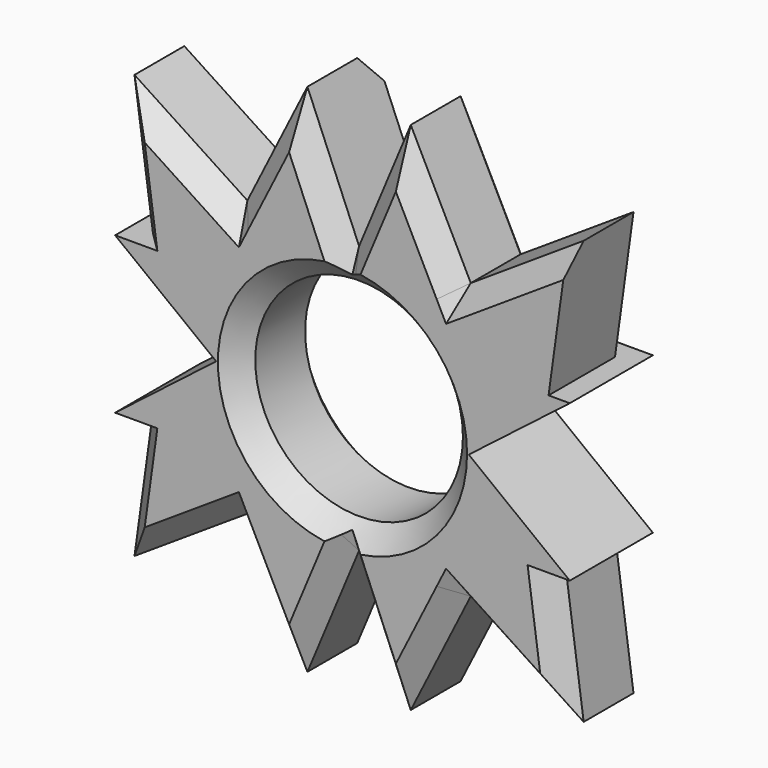
from build123d import *

# Parameters (mm, degrees)
F0_R          = 25.4053922475
F1_DEPTH      = 25.4
F2_SIZE       = 5.08
F3_T4_DEPTH   = 58.8942991577
F3_T9_DEPTH   = 59.1482991577
F3_T14_DEPTH  = 59.1482991577
F3_T19_DEPTH  = 59.1482991577
F3_T24_DEPTH  = 59.1482991577
F3_T29_DEPTH  = 58.8942991577
F3_T34_DEPTH  = 58.8942991577
F3_T39_DEPTH  = 58.8942991577
F3_T44_DEPTH  = 58.8942991577
F3_T49_DEPTH  = 59.1482991577
F3_T54_DEPTH  = 59.1482991577
F3_T59_DEPTH  = 58.8942991577
F3_T64_DEPTH  = 58.8942991577
F3_T69_DEPTH  = 59.1482991577
F3_T74_DEPTH  = 59.1482991577
F3_T79_DEPTH  = 59.1482991577
F3_T84_DEPTH  = 59.1482991577
F3_T89_DEPTH  = 58.8942991577
F3_T94_DEPTH  = 58.8942991577
F3_T99_DEPTH  = 58.8942991577
F3_T104_DEPTH = 59.1482991577
F3_T109_DEPTH = 59.1482991577
F3_T114_DEPTH = 59.1482991577
F3_T119_DEPTH = 58.8942991577
F3_T124_DEPTH = 59.1482991577
F3_T129_DEPTH = 59.1482991577
F3_T134_DEPTH = 58.8942991577
F3_T139_DEPTH = 58.8942991577
F3_T144_DEPTH = 58.8942991577
F3_T149_DEPTH = 58.8942991577


# Not quite as in the source:
# - a fillet or chamfer that OpenCascade refuses, or shapes differently, is made with other operations: its cross-section is extruded or revolved along the edge and cut away or added


with BuildPart() as f1:
    # F0 (on Front) → F1 (new body)
    with BuildSketch(Plane.XZ):
        Polygon((-55.6186027825, 19.1091839224), (-30.8941560641, 0), (-50.4200380058, 19.1091839224), align=None)
        Polygon((-54.9483810148, 51.8172029635), (-50.4200380058, 19.1091839224), (-27.3260947604, 33.7249476569), align=None)
        Polygon((-12.64267964, 63.0167225502), (-27.3260947604, 33.7249476569), (0, 32.7880373733), align=None)
        Polygon((12.64267964, 63.0167225502), (0, 32.7880373733), (27.3260947604, 33.7249476569), align=None)
        Polygon((54.9483810148, 51.8172029635), (27.3260947604, 33.7249476569), (50.4200380058, 19.1091839224), align=None)
        Polygon((55.6186027825, 19.1091839224), (50.4200380058, 19.1091839224), (30.8941560641, 0), align=None)
        Polygon((0, -32.7880373733), (-27.3260947604, -33.7249476569), (-12.64267964, -63.0167225502), align=None)
        Polygon((-27.3260947604, -33.7249476569), (-50.4200380058, -19.1091839224), (-54.9483810148, -51.8172029635), align=None)
        Polygon((-50.4200380058, -19.1091839224), (-30.8941560641, 0), (-55.6186027825, -19.1091839224), align=None)
        Polygon((27.3260947604, -33.7249476569), (0, -32.7880373733), (12.64267964, -63.0167225502), align=None)
        Polygon((50.4200380058, -19.1091839224), (27.3260947604, -33.7249476569), (54.9483810148, -51.8172029635), align=None)
        Polygon((30.8941560641, 0), (50.4200380058, -19.1091839224), (55.6186027825, -19.1091839224), align=None)
        Polygon((-50.4200380058, 19.1091839224), (-30.8941560641, 0), (-50.4200380058, -19.1091839224), (-27.3260947604, -33.7249476569), (0, -32.7880373733), (27.3260947604, -33.7249476569), (50.4200380058, -19.1091839224), (30.8941560641, 0), (50.4200380058, 19.1091839224), (27.3260947604, 33.7249476569), (0, 32.7880373733), (-27.3260947604, 33.7249476569), align=None)
        Circle(F0_R, mode=Mode.SUBTRACT)
    extrude(amount=F1_DEPTH)

    # F2
    f2_edges = [f1.edges().sort_by_distance(p)[0] for p in [
        (-25.405392, 0, 0),
        (-25.405392, -25.4, 0),
    ]]
    chamfer(f2_edges, length=F2_SIZE)

    # F3: chamfer of 5.08 on 30 edges, made by hand


with BuildPart() as f3_tool2:
    # F3_s3 → F3_t4 (new body)
    with BuildSketch(Plane(origin=(28.5608965027, 0, 56.9758018995), x_dir=(0, 1, 0), z_dir=(-0.4481296197, 0, -0.8939685922))):
        Polygon((0, -34.4618184336), (-5.08, -39.5418184336), (0, -39.5418184336), align=None)
    extrude(amount=F3_T4_DEPTH)

    split(bisect_by=Plane(origin=(2.2353786575, 4.079767946, 3.4128563917), x_dir=(-0.8769857612, 0.4805163626, 0), z_dir=(0.3874365964, 0.7071067812, 0.5915174416)), keep=Keep.TOP)


with BuildPart() as f1_1:
    add(f1.part)

    # F3_t1: cut F3_tool2
    add(f3_tool2.part, mode=Mode.SUBTRACT)


with BuildPart() as f3_tool7:
    # F3_s8 → F3_t9 (new body)
    with BuildSketch(Plane(origin=(-23.6516969458, 0, 15.4915684979), x_dir=(0, 1, 0), z_dir=(-0.8365319883, 0, 0.5479180892))):
        Polygon((0, -8.159535892), (-5.08, -13.239535892), (0, -13.239535892), align=None)
    extrude(amount=F3_T9_DEPTH)

    split(bisect_by=Plane(origin=(-15.4038916556, 17.2309092168, 7.7216807951), x_dir=(-0.7455258584, -0.6664767021, 0), z_dir=(-0.6321312537, 0.7071067812, 0.316875493)), keep=Keep.TOP)


with BuildPart() as f1_2:
    add(f1_1.part)

    # F3_t6: cut F3_tool7
    add(f3_tool7.part, mode=Mode.SUBTRACT)


with BuildPart() as f3_tool12:
    # F3_s13 → F3_t14 (new body)
    with BuildSketch(Plane(origin=(-9.8640749157, 0, 71.247771982), x_dir=(0, 1, 0), z_dir=(0.1371394006, 0, -0.9905517578))):
        Polygon((0, -42.2430352429), (-5.08, -47.3230352429), (0, -47.3230352429), align=None)
    extrude(amount=F3_T14_DEPTH)

    split(bisect_by=Plane.XY.offset(19.1091839224), keep=Keep.TOP)


with BuildPart() as f1_3:
    add(f1_2.part)

    # F3_t11: cut F3_tool12
    add(f3_tool12.part, mode=Mode.SUBTRACT)


with BuildPart() as f3_tool17:
    # F3_s18 → F3_t19 (new body)
    with BuildSketch(Plane(origin=(-1.7525126205, 0, -12.658320283), x_dir=(0, 1, 0), z_dir=(-0.1371394006, 0, -0.9905517578))):
        Polygon((0, -42.2430352429), (-5.08, -47.3230352429), (0, -47.3230352429), align=None)
    extrude(amount=F3_T19_DEPTH)

    split(bisect_by=Plane.XY.offset(-19.1091839224), keep=Keep.BOTTOM)


with BuildPart() as f1_4:
    add(f1_3.part)

    # F3_t16: cut F3_tool17
    add(f3_tool17.part, mode=Mode.SUBTRACT)


with BuildPart() as f3_tool22:
    # F3_s23 → F3_t24 (new body)
    with BuildSketch(Plane(origin=(-73.1311412461, 0, -47.8999915541), x_dir=(0, 1, 0), z_dir=(0.8365319883, 0, 0.5479180892))):
        Polygon((0, -8.159535892), (-5.08, -13.239535892), (0, -13.239535892), align=None)
    extrude(amount=F3_T24_DEPTH)

    split(bisect_by=Plane(origin=(-15.4038916556, 17.2309092168, -7.7216807951), x_dir=(-0.7455258584, -0.6664767021, 0), z_dir=(-0.6321312537, 0.7071067812, -0.316875493)), keep=Keep.TOP)


with BuildPart() as f1_5:
    add(f1_4.part)

    # F3_t21: cut F3_tool22
    add(f3_tool22.part, mode=Mode.SUBTRACT)


with BuildPart() as f3_tool27:
    # F3_s28 → F3_t29 (new body)
    with BuildSketch(Plane(origin=(2.1686166163, 0, -4.3261481905), x_dir=(0, 1, 0), z_dir=(0.4481296197, 0, -0.8939685922))):
        Polygon((0, -34.4618184336), (-5.08, -39.5418184336), (0, -39.5418184336), align=None)
    extrude(amount=F3_T29_DEPTH)

    split(bisect_by=Plane(origin=(2.2353786575, 4.079767946, -3.4128563917), x_dir=(-0.8769857612, 0.4805163626, 0), z_dir=(0.3874365964, 0.7071067812, -0.5915174416)), keep=Keep.TOP)


with BuildPart() as f1_6:
    add(f1_5.part)

    # F3_t26: cut F3_tool27
    add(f3_tool27.part, mode=Mode.SUBTRACT)


with BuildPart() as f3_tool32:
    # F3_s33 → F3_t34 (new body)
    with BuildSketch(Plane(origin=(-29.3549569097, 0, -70.1877905691), x_dir=(0, 1, 0), z_dir=(0.3858475139, 0, 0.9225625703))):
        Polygon((0, -7.5711827057), (-5.08, -12.6511827057), (0, -12.6511827057), align=None)
    extrude(amount=F3_T34_DEPTH)

    split(bisect_by=Plane(origin=(-3.4924448884, 3.7855913528, -1.4606610121), x_dir=(-0.7349918349, -0.6780759564, 0), z_dir=(-0.6523502495, 0.7071067812, -0.2728353936)), keep=Keep.TOP)


with BuildPart() as f1_7:
    add(f1_6.part)

    # F3_t31: cut F3_tool32
    add(f3_tool32.part, mode=Mode.SUBTRACT)


with BuildPart() as f3_tool37:
    # F3_s38 → F3_t39 (new body)
    with BuildSketch(Plane(origin=(6.6307379976, 0, -15.854114565), x_dir=(0, 1, 0), z_dir=(0.3858475139, 0, -0.9225625703))):
        Polygon((0, -7.5711827057), (-5.08, -12.6511827057), (0, -12.6511827057), align=None)
    extrude(amount=F3_T39_DEPTH)

    split(bisect_by=Plane(origin=(3.4924448884, 3.7855913528, -1.4606610121), x_dir=(-0.7349918349, 0.6780759564, 0), z_dir=(0.6523502495, 0.7071067812, -0.2728353936)), keep=Keep.TOP)


with BuildPart() as f1_8:
    add(f1_7.part)

    # F3_t36: cut F3_tool37
    add(f3_tool37.part, mode=Mode.SUBTRACT)


with BuildPart() as f3_tool42:
    # F3_s43 → F3_t44 (new body)
    with BuildSketch(Plane(origin=(-28.5608965027, 0, -56.9758018995), x_dir=(0, 1, 0), z_dir=(0.4481296197, 0, 0.8939685922))):
        Polygon((0, -34.4618184336), (-5.08, -39.5418184336), (0, -39.5418184336), align=None)
    extrude(amount=F3_T44_DEPTH)

    split(bisect_by=Plane(origin=(-2.2353786575, 4.079767946, -3.4128563917), x_dir=(-0.8769857612, -0.4805163626, 0), z_dir=(-0.3874365964, 0.7071067812, -0.5915174416)), keep=Keep.TOP)


with BuildPart() as f1_9:
    add(f1_8.part)

    # F3_t41: cut F3_tool42
    add(f3_tool42.part, mode=Mode.SUBTRACT)


with BuildPart() as f3_tool47:
    # F3_s48 → F3_t49 (new body)
    with BuildSketch(Plane(origin=(23.6516969458, 0, -15.4915684979), x_dir=(0, 1, 0), z_dir=(0.8365319883, 0, -0.5479180892))):
        Polygon((0, -8.159535892), (-5.08, -13.239535892), (0, -13.239535892), align=None)
    extrude(amount=F3_T49_DEPTH)

    split(bisect_by=Plane(origin=(15.4038916556, 17.2309092168, -7.7216807951), x_dir=(-0.7455258584, 0.6664767021, 0), z_dir=(0.6321312537, 0.7071067812, -0.316875493)), keep=Keep.TOP)


with BuildPart() as f1_10:
    add(f1_9.part)

    # F3_t46: cut F3_tool47
    add(f3_tool47.part, mode=Mode.SUBTRACT)


with BuildPart() as f3_tool52:
    # F3_s53 → F3_t54 (new body)
    with BuildSketch(Plane(origin=(9.8640749157, 0, -71.247771982), x_dir=(0, 1, 0), z_dir=(-0.1371394006, 0, 0.9905517578))):
        Polygon((0, -42.2430352429), (-5.08, -47.3230352429), (0, -47.3230352429), align=None)
    extrude(amount=F3_T54_DEPTH)

    split(bisect_by=Plane.XY.offset(-19.1091839224), keep=Keep.BOTTOM)


with BuildPart() as f1_11:
    add(f1_10.part)

    # F3_t51: cut F3_tool52
    add(f3_tool52.part, mode=Mode.SUBTRACT)


with BuildPart() as f3_tool57:
    # F3_s58 → F3_t59 (new body)
    with BuildSketch(Plane(origin=(29.3549569097, 0, 70.1877905691), x_dir=(0, 1, 0), z_dir=(-0.3858475139, 0, -0.9225625703))):
        Polygon((0, -7.5711827057), (-5.08, -12.6511827057), (0, -12.6511827057), align=None)
    extrude(amount=F3_T59_DEPTH)

    split(bisect_by=Plane(origin=(11.6715076337, 0, 4.8814273947), x_dir=(0, 1, 0), z_dir=(0.9225625703, 0, 0.3858475139)), keep=Keep.TOP)


with BuildPart() as f1_12:
    add(f1_11.part)

    # F3_t56: cut F3_tool57
    add(f3_tool57.part, mode=Mode.SUBTRACT)


with BuildPart() as f3_tool62:
    # F3_s63 → F3_t64 (new body)
    with BuildSketch(Plane(origin=(-2.1686166163, 0, 4.3261481905), x_dir=(0, 1, 0), z_dir=(-0.4481296197, 0, 0.8939685922))):
        Polygon((0, -34.4618184336), (-5.08, -39.5418184336), (0, -39.5418184336), align=None)
    extrude(amount=F3_T64_DEPTH)

    split(bisect_by=Plane(origin=(-2.2353786575, 4.079767946, 3.4128563917), x_dir=(-0.8769857612, -0.4805163626, 0), z_dir=(-0.3874365964, 0.7071067812, 0.5915174416)), keep=Keep.TOP)


with BuildPart() as f1_13:
    add(f1_12.part)

    # F3_t61: cut F3_tool62
    add(f3_tool62.part, mode=Mode.SUBTRACT)


with BuildPart() as f3_tool67:
    # F3_s68 → F3_t69 (new body)
    with BuildSketch(Plane(origin=(73.1311412461, 0, 47.8999915541), x_dir=(0, 1, 0), z_dir=(-0.8365319883, 0, -0.5479180892))):
        Polygon((0, -8.159535892), (-5.08, -13.239535892), (0, -13.239535892), align=None)
    extrude(amount=F3_T69_DEPTH)

    split(bisect_by=Plane(origin=(15.4038916556, 17.2309092168, 7.7216807951), x_dir=(-0.7455258584, 0.6664767021, 0), z_dir=(0.6321312537, 0.7071067812, 0.316875493)), keep=Keep.TOP)


with BuildPart() as f1_14:
    add(f1_13.part)

    # F3_t66: cut F3_tool67
    add(f3_tool67.part, mode=Mode.SUBTRACT)


with BuildPart() as f3_tool72:
    # F3_s73 → F3_t74 (new body)
    with BuildSketch(Plane(origin=(1.7525126205, 0, 12.658320283), x_dir=(0, 1, 0), z_dir=(0.1371394006, 0, 0.9905517578))):
        Polygon((0, -42.2430352429), (-5.08, -47.3230352429), (0, -47.3230352429), align=None)
    extrude(amount=F3_T74_DEPTH)

    split(bisect_by=Plane.XY.offset(19.1091839224), keep=Keep.TOP)


with BuildPart() as f1_15:
    add(f1_14.part)

    # F3_t71: cut F3_tool72
    add(f3_tool72.part, mode=Mode.SUBTRACT)


with BuildPart() as f3_tool77:
    # F3_s78 → F3_t79 (new body)
    with BuildSketch(Plane(origin=(-9.8640749157, 0, 71.247771982), x_dir=(0, 1, 0), z_dir=(0.1371394006, 0, -0.9905517578))):
        Polygon((-25.4, -42.2430352429), (-20.32, -47.3230352429), (-25.4, -47.3230352429), align=None)
    extrude(amount=F3_T79_DEPTH)

    split(bisect_by=Plane.XY.offset(19.1091839224), keep=Keep.TOP)


with BuildPart() as f1_16:
    add(f1_15.part)

    # F3_t76: cut F3_tool77
    add(f3_tool77.part, mode=Mode.SUBTRACT)


with BuildPart() as f3_tool82:
    # F3_s83 → F3_t84 (new body)
    with BuildSketch(Plane(origin=(-23.6516969458, 0, 15.4915684979), x_dir=(0, 1, 0), z_dir=(-0.8365319883, 0, 0.5479180892))):
        Polygon((-25.4, -8.159535892), (-20.32, -13.239535892), (-25.4, -13.239535892), align=None)
    extrude(amount=F3_T84_DEPTH)

    split(bisect_by=Plane(origin=(-26.757292777, -29.9309092168, 13.4129269658), x_dir=(0.7455258584, -0.6664767021, 0), z_dir=(-0.6321312537, -0.7071067812, 0.316875493)), keep=Keep.TOP)


with BuildPart() as f1_17:
    add(f1_16.part)

    # F3_t81: cut F3_tool82
    add(f3_tool82.part, mode=Mode.SUBTRACT)


with BuildPart() as f3_tool87:
    # F3_s88 → F3_t89 (new body)
    with BuildSketch(Plane(origin=(28.5608965027, 0, 56.9758018995), x_dir=(0, 1, 0), z_dir=(-0.4481296197, 0, -0.8939685922))):
        Polygon((-25.4, -34.4618184336), (-20.32, -39.5418184336), (-25.4, -39.5418184336), align=None)
    extrude(amount=F3_T89_DEPTH)

    split(bisect_by=Plane(origin=(9.1939383908, -16.779767946, 14.0368126434), x_dir=(0.8769857612, 0.4805163626, 0), z_dir=(0.3874365964, -0.7071067812, 0.5915174416)), keep=Keep.TOP)


with BuildPart() as f1_18:
    add(f1_17.part)

    # F3_t86: cut F3_tool87
    add(f3_tool87.part, mode=Mode.SUBTRACT)


with BuildPart() as f3_tool92:
    # F3_s93 → F3_t94 (new body)
    with BuildSketch(Plane(origin=(-6.6307379976, 0, 15.854114565), x_dir=(0, 1, 0), z_dir=(-0.3858475139, 0, 0.9225625703))):
        Polygon((-25.4, -7.5711827057), (-20.32, -12.6511827057), (-25.4, -12.6511827057), align=None)
    extrude(amount=F3_T94_DEPTH)

    split(bisect_by=Plane(origin=(-15.2089895306, -16.4855913528, 6.3609244384), x_dir=(0.7349918349, -0.6780759564, 0), z_dir=(-0.6523502495, -0.7071067812, 0.2728353936)), keep=Keep.TOP)


with BuildPart() as f1_19:
    add(f1_18.part)

    # F3_t91: cut F3_tool92
    add(f3_tool92.part, mode=Mode.SUBTRACT)


with BuildPart() as f3_tool97:
    # F3_s98 → F3_t99 (new body)
    with BuildSketch(Plane(origin=(29.3549569097, 0, 70.1877905691), x_dir=(0, 1, 0), z_dir=(-0.3858475139, 0, -0.9225625703))):
        Polygon((-25.4, -7.5711827057), (-20.32, -12.6511827057), (-25.4, -12.6511827057), align=None)
    extrude(amount=F3_T99_DEPTH)

    split(bisect_by=Plane(origin=(15.2089895306, -16.4855913528, 6.3609244384), x_dir=(0.7349918349, 0.6780759564, 0), z_dir=(0.6523502495, -0.7071067812, 0.2728353936)), keep=Keep.TOP)


with BuildPart() as f1_20:
    add(f1_19.part)

    # F3_t96: cut F3_tool97
    add(f3_tool97.part, mode=Mode.SUBTRACT)


with BuildPart() as f3_tool102:
    # F3_s103 → F3_t104 (new body)
    with BuildSketch(Plane(origin=(73.1311412461, 0, 47.8999915541), x_dir=(0, 1, 0), z_dir=(-0.8365319883, 0, -0.5479180892))):
        Polygon((-25.4, -8.159535892), (-20.32, -13.239535892), (-25.4, -13.239535892), align=None)
    extrude(amount=F3_T104_DEPTH)

    split(bisect_by=Plane(origin=(26.757292777, -29.9309092168, 13.4129269658), x_dir=(0.7455258584, 0.6664767021, 0), z_dir=(0.6321312537, -0.7071067812, 0.316875493)), keep=Keep.TOP)


with BuildPart() as f1_21:
    add(f1_20.part)

    # F3_t101: cut F3_tool102
    add(f3_tool102.part, mode=Mode.SUBTRACT)


with BuildPart() as f3_tool107:
    # F3_s108 → F3_t109 (new body)
    with BuildSketch(Plane(origin=(9.8640749157, 0, -71.247771982), x_dir=(0, 1, 0), z_dir=(-0.1371394006, 0, 0.9905517578))):
        Polygon((-25.4, -42.2430352429), (-20.32, -47.3230352429), (-25.4, -47.3230352429), align=None)
    extrude(amount=F3_T109_DEPTH)

    split(bisect_by=Plane.XY.offset(-19.1091839224), keep=Keep.BOTTOM)


with BuildPart() as f1_22:
    add(f1_21.part)

    # F3_t106: cut F3_tool107
    add(f3_tool107.part, mode=Mode.SUBTRACT)


with BuildPart() as f3_tool112:
    # F3_s113 → F3_t114 (new body)
    with BuildSketch(Plane(origin=(23.6516969458, 0, -15.4915684979), x_dir=(0, 1, 0), z_dir=(0.8365319883, 0, -0.5479180892))):
        Polygon((-25.4, -8.159535892), (-20.32, -13.239535892), (-25.4, -13.239535892), align=None)
    extrude(amount=F3_T114_DEPTH)

    split(bisect_by=Plane(origin=(26.757292777, -29.9309092168, -13.4129269658), x_dir=(0.7455258584, 0.6664767021, 0), z_dir=(0.6321312537, -0.7071067812, -0.316875493)), keep=Keep.TOP)


with BuildPart() as f1_23:
    add(f1_22.part)

    # F3_t111: cut F3_tool112
    add(f3_tool112.part, mode=Mode.SUBTRACT)


with BuildPart() as f3_tool117:
    # F3_s118 → F3_t119 (new body)
    with BuildSketch(Plane(origin=(-2.1686166163, 0, 4.3261481905), x_dir=(0, 1, 0), z_dir=(-0.4481296197, 0, 0.8939685922))):
        Polygon((-25.4, -34.4618184336), (-20.32, -39.5418184336), (-25.4, -39.5418184336), align=None)
    extrude(amount=F3_T119_DEPTH)

    split(bisect_by=Plane(origin=(-9.1939383908, -16.779767946, 14.0368126434), x_dir=(0.8769857612, -0.4805163626, 0), z_dir=(-0.3874365964, -0.7071067812, 0.5915174416)), keep=Keep.TOP)


with BuildPart() as f1_24:
    add(f1_23.part)

    # F3_t116: cut F3_tool117
    add(f3_tool117.part, mode=Mode.SUBTRACT)


with BuildPart() as f3_tool122:
    # F3_s123 → F3_t124 (new body)
    with BuildSketch(Plane(origin=(-1.7525126205, 0, -12.658320283), x_dir=(0, 1, 0), z_dir=(-0.1371394006, 0, -0.9905517578))):
        Polygon((-25.4, -42.2430352429), (-20.32, -47.3230352429), (-25.4, -47.3230352429), align=None)
    extrude(amount=F3_T124_DEPTH)

    split(bisect_by=Plane.XY.offset(-19.1091839224), keep=Keep.BOTTOM)


with BuildPart() as f1_25:
    add(f1_24.part)

    # F3_t121: cut F3_tool122
    add(f3_tool122.part, mode=Mode.SUBTRACT)


with BuildPart() as f3_tool127:
    # F3_s128 → F3_t129 (new body)
    with BuildSketch(Plane(origin=(-73.1311412461, 0, -47.8999915541), x_dir=(0, 1, 0), z_dir=(0.8365319883, 0, 0.5479180892))):
        Polygon((-25.4, -8.159535892), (-20.32, -13.239535892), (-25.4, -13.239535892), align=None)
    extrude(amount=F3_T129_DEPTH)

    split(bisect_by=Plane(origin=(-26.757292777, -29.9309092168, -13.4129269658), x_dir=(0.7455258584, -0.6664767021, 0), z_dir=(-0.6321312537, -0.7071067812, -0.316875493)), keep=Keep.TOP)


with BuildPart() as f1_26:
    add(f1_25.part)

    # F3_t126: cut F3_tool127
    add(f3_tool127.part, mode=Mode.SUBTRACT)


with BuildPart() as f3_tool132:
    # F3_s133 → F3_t134 (new body)
    with BuildSketch(Plane(origin=(2.1686166163, 0, -4.3261481905), x_dir=(0, 1, 0), z_dir=(0.4481296197, 0, -0.8939685922))):
        Polygon((-25.4, -34.4618184336), (-20.32, -39.5418184336), (-25.4, -39.5418184336), align=None)
    extrude(amount=F3_T134_DEPTH)

    split(bisect_by=Plane(origin=(9.1939383908, -16.779767946, -14.0368126434), x_dir=(0.8769857612, 0.4805163626, 0), z_dir=(0.3874365964, -0.7071067812, -0.5915174416)), keep=Keep.TOP)


with BuildPart() as f1_27:
    add(f1_26.part)

    # F3_t131: cut F3_tool132
    add(f3_tool132.part, mode=Mode.SUBTRACT)


with BuildPart() as f3_tool137:
    # F3_s138 → F3_t139 (new body)
    with BuildSketch(Plane(origin=(6.6307379976, 0, -15.854114565), x_dir=(0, 1, 0), z_dir=(0.3858475139, 0, -0.9225625703))):
        Polygon((-25.4, -7.5711827057), (-20.32, -12.6511827057), (-25.4, -12.6511827057), align=None)
    extrude(amount=F3_T139_DEPTH)

    split(bisect_by=Plane(origin=(15.2089895306, -16.4855913528, -6.3609244384), x_dir=(0.7349918349, 0.6780759564, 0), z_dir=(0.6523502495, -0.7071067812, -0.2728353936)), keep=Keep.TOP)


with BuildPart() as f1_28:
    add(f1_27.part)

    # F3_t136: cut F3_tool137
    add(f3_tool137.part, mode=Mode.SUBTRACT)


with BuildPart() as f3_tool142:
    # F3_s143 → F3_t144 (new body)
    with BuildSketch(Plane(origin=(-28.5608965027, 0, -56.9758018995), x_dir=(0, 1, 0), z_dir=(0.4481296197, 0, 0.8939685922))):
        Polygon((-25.4, -34.4618184336), (-20.32, -39.5418184336), (-25.4, -39.5418184336), align=None)
    extrude(amount=F3_T144_DEPTH)

    split(bisect_by=Plane(origin=(-9.1939383908, -16.779767946, -14.0368126434), x_dir=(0.8769857612, -0.4805163626, 0), z_dir=(-0.3874365964, -0.7071067812, -0.5915174416)), keep=Keep.TOP)


with BuildPart() as f1_29:
    add(f1_28.part)

    # F3_t141: cut F3_tool142
    add(f3_tool142.part, mode=Mode.SUBTRACT)


with BuildPart() as f3_tool147:
    # F3_s148 → F3_t149 (new body)
    with BuildSketch(Plane(origin=(-29.3549569097, 0, -70.1877905691), x_dir=(0, 1, 0), z_dir=(0.3858475139, 0, 0.9225625703))):
        Polygon((-25.4, -7.5711827057), (-20.32, -12.6511827057), (-25.4, -12.6511827057), align=None)
    extrude(amount=F3_T149_DEPTH)

    split(bisect_by=Plane(origin=(-15.2089895306, -16.4855913528, -6.3609244384), x_dir=(0.7349918349, -0.6780759564, 0), z_dir=(-0.6523502495, -0.7071067812, -0.2728353936)), keep=Keep.TOP)


with BuildPart() as f1_30:
    add(f1_29.part)

    # F3_t146: cut F3_tool147
    add(f3_tool147.part, mode=Mode.SUBTRACT)


solid = f1_30.part
